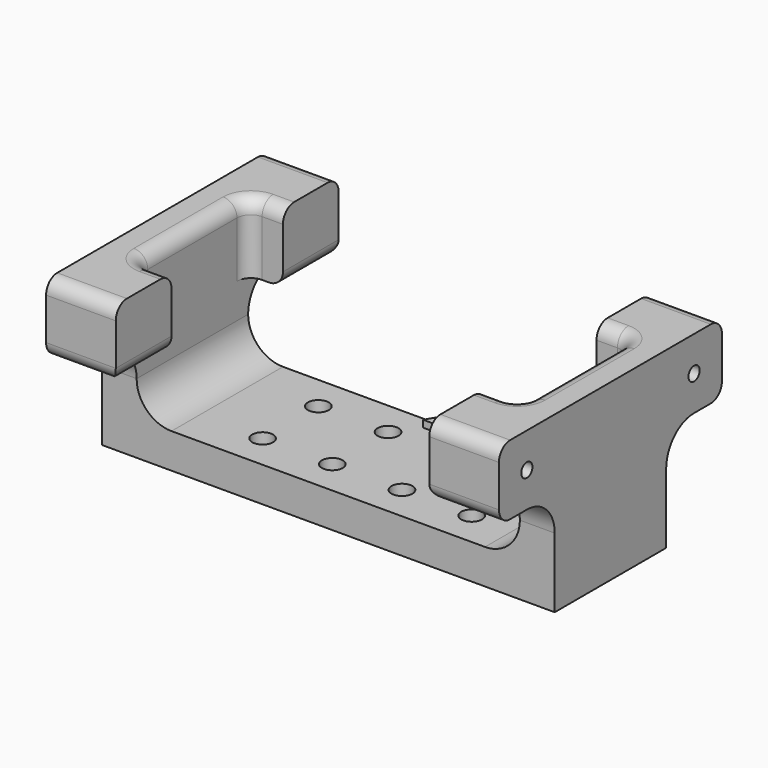
from build123d import *

# Parameters (mm, degrees)
F1_DEPTH    = 10
F4_DEPTH    = 1
F5_W        = 10
F5_H        = 10.0000003353
F6_DEPTH    = 10
F7_D        = 2
F7_DEPTH    = 8
F7_TIP      = 0.600860619
F8_R        = 2
F9_T1_DEPTH = 5
F9_T3_DEPTH = 20
F10_R       = 2
F12_D       = 3
F13_R       = 2


# Not quite as in the source:
# - a fillet or chamfer that OpenCascade refuses, or shapes differently, is made with other operations: its cross-section is extruded or revolved along the edge and cut away or added


with BuildPart() as f1:
    # F0 (on Front) → F1 (new body, symmetric)
    with BuildSketch(Plane.XZ):
        Polygon((-27.5, 25), (-32.5, 25), (-32.5, 0), (32.5, 0), (32.5, 25), (27.5, 25), (27.5, 5), (-27.5, 5), align=None)
    extrude(amount=F1_DEPTH, both=True)

    # F3 (on face) → F4 (join)
    with BuildSketch(Plane.XY.offset(5)):
        Polygon((1, 8.2679491924), (0, 10), (-1, 8.2679491924), align=None)
    extrude(amount=F4_DEPTH)

    # F5 (on face) → F6 (join)
    with BuildSketch(Plane(origin=(-32.5, 0, 0), x_dir=(0, -1, 0), z_dir=(-1, 0, 0))):
        with Locations((-15, 19.9999998324)):
            Rectangle(F5_W, F5_H)
        with Locations((15, 19.9999998324)):
            Rectangle(F5_W, F5_H)
    extrude(amount=-F6_DEPTH)

    # F7
    with Locations(Plane(origin=(-32.5, 0, 0), x_dir=(0, -1, 0), z_dir=(-1, 0, 0))):
        with Locations((-15, 19.9999998324), (15, 19.9999998324)):
            Hole(F7_D / 2, depth=F7_DEPTH)
            with Locations((0, 0, -(F7_DEPTH + F7_TIP / 2))):  # 118° drill point
                Cone(0, F7_D / 2, F7_TIP, mode=Mode.SUBTRACT)

    # F8
    f8_edges = [f1.edges().sort_by_distance(p)[0] for p in [
        (-27.5, -20, 25),
        (-27.5, 20, 25),
        (-27.5, 20, 15),
        (-22.5, 15, 15),
        (-22.5, -15, 15),
        (-27.5, -20, 15),
    ]]
    fillet(f8_edges, radius=F8_R)

    # F9: fillet of radius 5 on 4 edges, made by hand

    # F9_s2 → F9_t1 (join)
    with BuildSketch(Plane.YZ.offset(-32.5)):
        with BuildLine():
            ThreePointArc((-15, 14.9999996647), (-11.4644660941, 13.5355335707), (-10, 9.9999996647))
            Line((-10, 9.9999996647), (-10, 14.9999996647))
            Line((-10, 14.9999996647), (-15, 14.9999996647))
        make_face()
        with BuildLine():
            ThreePointArc((15, 14.9999996647), (11.4644660941, 13.5355335707), (10, 9.9999996647))
            Line((10, 9.9999996647), (10, 14.9999996647))
            Line((10, 14.9999996647), (15, 14.9999996647))
        make_face()
    extrude(amount=F9_T1_DEPTH)

    # F9_s4 → F9_t3 (join)
    with BuildSketch(Plane.XZ.offset(-10)):
        with BuildLine():
            ThreePointArc((-27.5, 10), (-26.0355339059, 6.4644660941), (-22.5, 5))
            Line((-22.5, 5), (-27.5, 5))
            Line((-27.5, 5), (-27.5, 10))
        make_face()
        with BuildLine():
            ThreePointArc((22.5, 5), (26.0355339059, 6.4644660941), (27.5, 10))
            Line((27.5, 10), (27.5, 5))
            Line((27.5, 5), (22.5, 5))
        make_face()
    extrude(amount=F9_T3_DEPTH)

    # F10
    f10_edges = [f1.edges().sort_by_distance(p)[0] for p in [
        (-27.5, 10, 20),
        (-27.5, -10, 20),
    ]]
    fillet(f10_edges, radius=F10_R)

    # F11: F1 across plane


with BuildPart() as f1_1:
    add(f1.part)
    add(f1.part.mirror(Plane.YZ))

    # F12 (through all)
    with Locations(Plane(origin=(0, 0, 0), x_dir=(1, 0, 0), z_dir=(0, 0, -1))):
        with Locations((-13.4210362619, 5.0000001118), (-3.4210362619, 5.0000001118), (6.5789637381, 5.0000001118), (16.5789637381, 5.0000001118), (-13.4210362619, -4.9999998882), (-3.4210362619, -4.9999998882), (6.5789637381, -4.9999998882), (16.5789637381, -4.9999998882)):
            Hole(F12_D / 2)

    # F13
    f13_edges = [f1_1.edges().sort_by_distance(p)[0] for p in [
        (-27.5, 0, 25),
        (27.5, 0, 25),
        (-24, -10, 25),
        (-26.914214, -9.414214, 25),
        (-26.914214, 9.414214, 25),
        (-24, 10, 25),
        (24, 10, 25),
        (26.914214, 9.414214, 25),
        (26.914214, -9.414214, 25),
        (24, -10, 25),
    ]]
    fillet(f13_edges, radius=F13_R)


solid = f1_1.part
